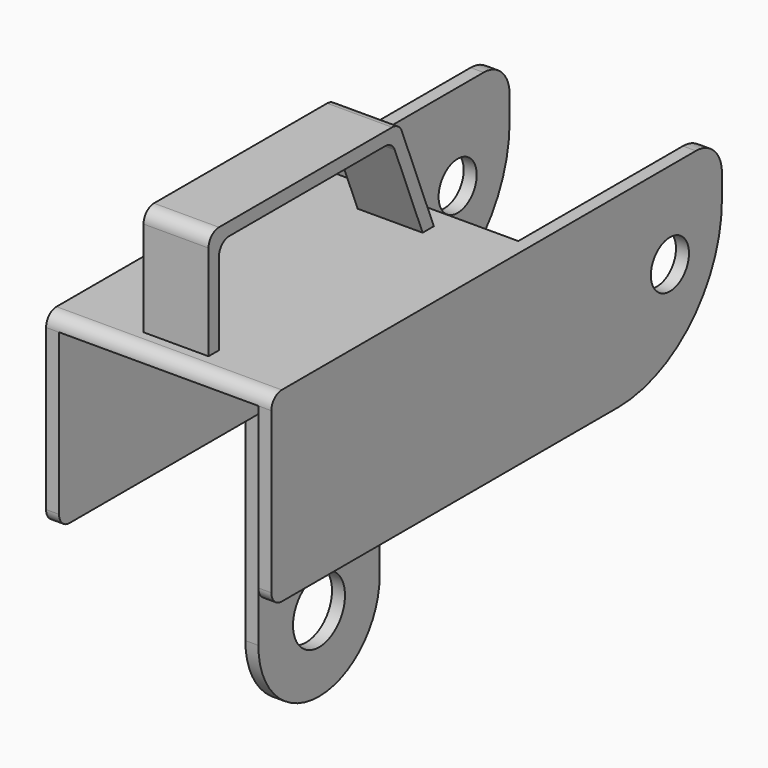
from build123d import *

# Parameters (mm, degrees)
F1_DEPTH = 65
F2_R     = 5.5
F3_DEPTH = 52.001
F4_W     = 46
F4_H     = 55
F5_DEPTH = 25
F7_DEPTH = 7.5
F8_R     = 7.5
F9_DEPTH = 3
F10_R    = 2.99999


# Not quite as in the source:
# - a fillet or chamfer is up to 0.001 mm smaller than in the source, because OpenCascade refuses the exact size
# - a feature names something its author has since deleted; it is built from what else it names


with BuildPart() as f1:
    # F0 (on Front) → F1 (new body, symmetric)
    with BuildSketch(Plane.XZ):
        Polygon((-23, 20), (23, 20), (23, -20), (26, -20), (26, 23), (-26, 23), (-26, -20), (-23, -20), align=None)
    extrude(amount=F1_DEPTH, both=True)

    # F2 (on face) → F3 (cut, through all)
    with BuildSketch(Plane.YZ.offset(26)):
        with Locations((50, 3)):
            Circle(F2_R)
        with BuildLine():
            Line((65, -20), (65, 10))
            ThreePointArc((65, 10), (56.2132034356, -11.2132034356), (35, -20))
            Line((35, -20), (65, -20))
        make_face()
        with BuildLine():
            ThreePointArc((63.1113759485, 20.4761893015), (64.5119654739, 18.161266652), (65, 15.5))
            Line((65, 15.5), (65, 23))
            Line((65, 23), (62.0370116692, 23))
            ThreePointArc((62.0370116692, 23), (62.6030536231, 21.7503800228), (63.1113759485, 20.4761893015))
        make_face()
        with BuildLine():
            ThreePointArc((57.5, 23), (60.5764086399, 22.3400080322), (63.1113759485, 20.4761893015))
            ThreePointArc((63.1113759485, 20.4761893015), (62.6030536231, 21.7503800228), (62.0370116692, 23))
            Line((62.0370116692, 23), (57.5, 23))
        make_face()
    extrude(amount=-F3_DEPTH, mode=Mode.SUBTRACT)

    # F4 (on face) → F5 (cut)
    with BuildSketch(Plane(origin=(0, 0, 20), x_dir=(1, 0, 0), z_dir=(0, 0, -1))):
        with Locations((0, -37.5)):
            Rectangle(F4_W, F4_H)
    extrude(amount=-F5_DEPTH, mode=Mode.SUBTRACT)

    # F6 (on Right) → F7 (join, symmetric)
    with BuildSketch(Plane.YZ):
        Polygon((-60, 48), (-60, 23), (-57, 23), (-57, 45), (-7.0310988843, 45), (1.7689011157, 23), (5, 23), (-5, 48), align=None)
    extrude(amount=F7_DEPTH, both=True)

    # F8 (on face) → F9 (join)
    with BuildSketch(Plane(origin=(-26, 0, 0), x_dir=(0, -1, 0), z_dir=(-1, 0, 0))):
        with BuildLine():
            Line((7.5, -20), (-27.5, -20))
            Line((-27.5, -20), (-27.5, -67))
            ThreePointArc((-27.5, -67), (-10, -49.5), (7.5, -67))
            Line((7.5, -67), (7.5, -20))
        make_face()
        with BuildLine():
            ThreePointArc((7.5, -67), (-10, -49.5), (-27.5, -67))
            ThreePointArc((-27.5, -67), (-10, -84.5), (7.5, -67))
        make_face()
        with Locations((-10, -67)):
            Circle(F8_R, mode=Mode.SUBTRACT)
    extrude(amount=-F9_DEPTH)

    # F10 (radius 3 in the source; OpenCascade refuses exactly that, so slightly less here)
    f10_edges = [f1.edges().sort_by_distance(p)[0] for p in [
        (24.5, -65, -20),
        (-24.5, -65, -20),
        (0, -60, 48),
        (0, -57, 45),
        (0, -7.031099, 45),
        (0, -5, 48),
        (0, -65, 23),
    ]]
    fillet(f10_edges, radius=F10_R)


solid = f1.part
